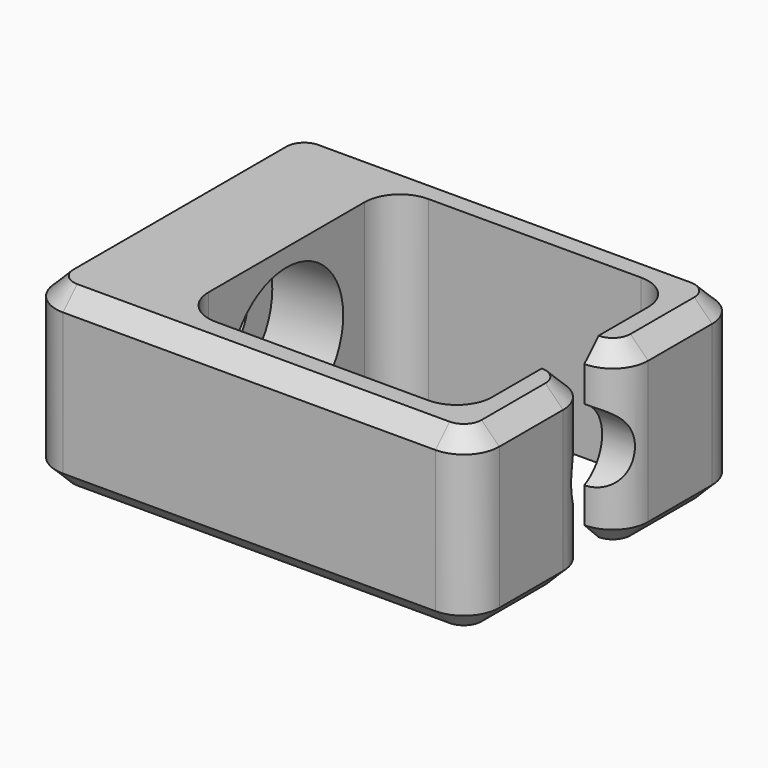
from build123d import *

# Parameters (mm, degrees)
F1_DEPTH    = 5
F2_R        = 2.25
F3_DEPTH    = 100
F4_R        = 4
F5_DEPTH    = 4
F6_T1_DEPTH = 10
F6_T3_DEPTH = 20
F6_T5_DEPTH = 12.9844355629
F6_T7_DEPTH = 12.9844355629
F7_SIZE     = 1


# Not quite as in the source:
# - a fillet or chamfer that OpenCascade refuses, or shapes differently, is made with other operations: its cross-section is extruded or revolved along the edge and cut away or added


with BuildPart() as f1:
    # F0 (on Top) → F1 (new body, symmetric)
    with BuildSketch(Plane.XY):
        Polygon((12.5, 1), (12.5, 9.5), (-12.5, 9.5), (-12.5, -9.5), (12.5, -9.5), (12.5, -1), (10.5, -1), (10.5, -7.5), (-5.5, -7.5), (-5.5, 7.5), (10.5, 7.5), (10.5, 1), align=None)
    extrude(amount=F1_DEPTH, both=True)

    # F2 (on face) → F3 (cut, symmetric)
    with BuildSketch(Plane.YZ.offset(-5.5)):
        Circle(F2_R)
    extrude(amount=F3_DEPTH, both=True, mode=Mode.SUBTRACT)

    # F4 (on face) → F5 (cut)
    with BuildSketch(Plane.YZ.offset(-5.5)):
        Circle(F4_R)
    extrude(amount=-F5_DEPTH, mode=Mode.SUBTRACT)

    # F6: fillet of radius 2 on 12 edges, made by hand

    # F6_s2 → F6_t1 (join)
    with BuildSketch(Plane.XY.offset(-5)):
        with BuildLine():
            ThreePointArc((10.5, -5.5), (9.9142135624, -6.9142135624), (8.5, -7.5))
            Line((8.5, -7.5), (10.5, -7.5))
            Line((10.5, -7.5), (10.5, -5.5))
        make_face()
        with BuildLine():
            ThreePointArc((10.5, 5.5), (9.9142135624, 6.9142135624), (8.5, 7.5))
            Line((8.5, 7.5), (10.5, 7.5))
            Line((10.5, 7.5), (10.5, 5.5))
        make_face()
        with BuildLine():
            ThreePointArc((-5.5, 5.5), (-4.9142135624, 6.9142135624), (-3.5, 7.5))
            Line((-3.5, 7.5), (-5.5, 7.5))
            Line((-5.5, 7.5), (-5.5, 5.5))
        make_face()
        with BuildLine():
            ThreePointArc((-3.5, -7.5), (-4.9142135624, -6.9142135624), (-5.5, -5.5))
            Line((-5.5, -5.5), (-5.5, -7.5))
            Line((-5.5, -7.5), (-3.5, -7.5))
        make_face()
    extrude(amount=F6_T1_DEPTH)

    # F6_s4 → F6_t3 (cut)
    with BuildSketch(Plane.XY.offset(-10)):
        with BuildLine():
            ThreePointArc((-10.5, 9.5), (-11.9142135624, 8.9142135624), (-12.5, 7.5))
            Line((-12.5, 7.5), (-12.5, 9.5))
            Line((-12.5, 9.5), (-10.5, 9.5))
        make_face()
        with BuildLine():
            ThreePointArc((-12.5, -7.5), (-11.9142135624, -8.9142135624), (-10.5, -9.5))
            Line((-10.5, -9.5), (-12.5, -9.5))
            Line((-12.5, -9.5), (-12.5, -7.5))
        make_face()
        with BuildLine():
            ThreePointArc((12.5, 7.5), (11.9142135624, 8.9142135624), (10.5, 9.5))
            Line((10.5, 9.5), (12.5, 9.5))
            Line((12.5, 9.5), (12.5, 7.5))
        make_face()
        with BuildLine():
            ThreePointArc((10.5, -9.5), (11.9142135624, -8.9142135624), (12.5, -7.5))
            Line((12.5, -7.5), (12.5, -9.5))
            Line((12.5, -9.5), (10.5, -9.5))
        make_face()
    extrude(amount=F6_T3_DEPTH, mode=Mode.SUBTRACT)

    # F6_s6 → F6_t5 (cut)
    with BuildSketch(Plane.XY.offset(-2.9844355629)):
        with BuildLine():
            ThreePointArc((12.5, -3), (11.9142135624, -1.5857864376), (10.5, -1))
            Line((10.5, -1), (12.5, -1))
            Line((12.5, -1), (12.5, -3))
        make_face()
        with BuildLine():
            ThreePointArc((12.5, 3), (11.9142135624, 1.5857864376), (10.5, 1))
            Line((10.5, 1), (12.5, 1))
            Line((12.5, 1), (12.5, 3))
        make_face()
    extrude(amount=F6_T5_DEPTH, mode=Mode.SUBTRACT)

    # F6_s8 → F6_t7 (cut)
    with BuildSketch(Plane.XY.offset(-10)):
        with BuildLine():
            ThreePointArc((12.5, -3), (11.9142135624, -1.5857864376), (10.5, -1))
            Line((10.5, -1), (12.5, -1))
            Line((12.5, -1), (12.5, -3))
        make_face()
        with BuildLine():
            ThreePointArc((12.5, 3), (11.9142135624, 1.5857864376), (10.5, 1))
            Line((10.5, 1), (12.5, 1))
            Line((12.5, 1), (12.5, 3))
        make_face()
    extrude(amount=F6_T7_DEPTH, mode=Mode.SUBTRACT)

    # F7
    f7_edges = [f1.edges().sort_by_distance(p)[0] for p in [
        (0, 9.5, 5),
        (-12.5, 0, -5),
    ]]
    chamfer(f7_edges, length=F7_SIZE)


solid = f1.part
